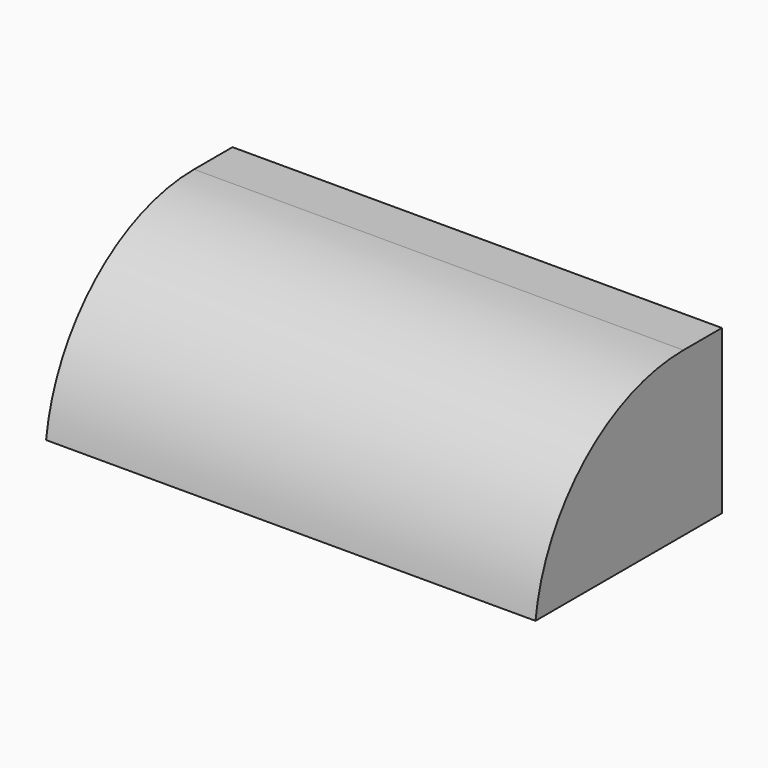
from build123d import *

# Parameters (mm, degrees)
F0_W        = 42
F0_H        = 20
F1_DEPTH    = 14
F2_T1_DEPTH = 121.3725393319
F3_T        = -1.1


# Not quite as in the source:
# - a fillet or chamfer that OpenCascade refuses, or shapes differently, is made with other operations: its cross-section is extruded or revolved along the edge and cut away or added


with BuildPart() as f1:
    # F0 (on Top) → F1 (new body)
    with BuildSketch(Plane.XY):
        Rectangle(F0_W, F0_H)
    extrude(amount=F1_DEPTH)

    # F2: fillet of radius 16 on 1 edges, made by hand

    # F2_s2 → F2_t1 (cut)
    with BuildSketch(Plane.YZ.offset(-60.686269666)):
        with BuildLine():
            ThreePointArc((-10, 0), (-4.7084973779, 10), (5.8745078664, 14))
            Line((5.8745078664, 14), (-10, 14))
            Line((-10, 14), (-10, 0))
        make_face()
    extrude(amount=F2_T1_DEPTH, mode=Mode.SUBTRACT)

    # F3
    f3_openings = [f1.faces().sort_by_distance(p)[0] for p in [
        (0, 10, 7),
        (0, 0, 0),
    ]]
    offset(amount=F3_T, openings=f3_openings)


solid = f1.part
